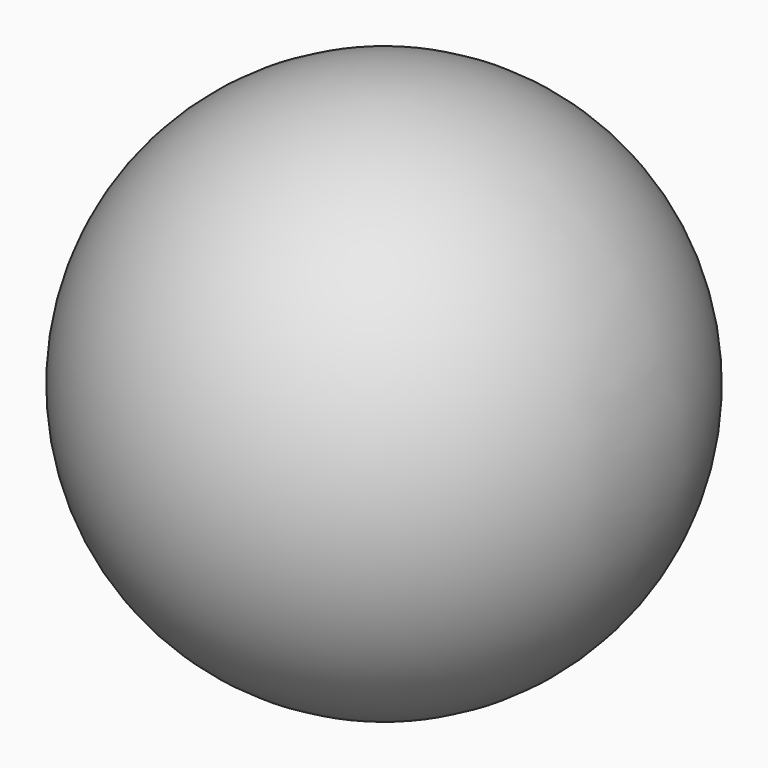
from build123d import *


# Not quite as in the source:
# - a feature names something its author has since deleted; it is built from what else it names


with BuildPart() as f1:
    # F0 (on Front) → F1 (revolve)
    with BuildSketch(Plane.XZ):
        with BuildLine():
            ThreePointArc((0, 44.6098931134), (22.3049465567, 22.3049465567), (0, 0))
            Line((0, 0), (0, -1.5948133343))
            ThreePointArc((0, -1.5948133343), (23.899759891, 22.3049465567), (0, 46.2047064477))
            Line((0, 46.2047064477), (0, 44.6098931134))
        make_face()
    revolve(axis=Axis((0, 0, 35.0403487682), (0, 0, 1)))


solid = f1.part
